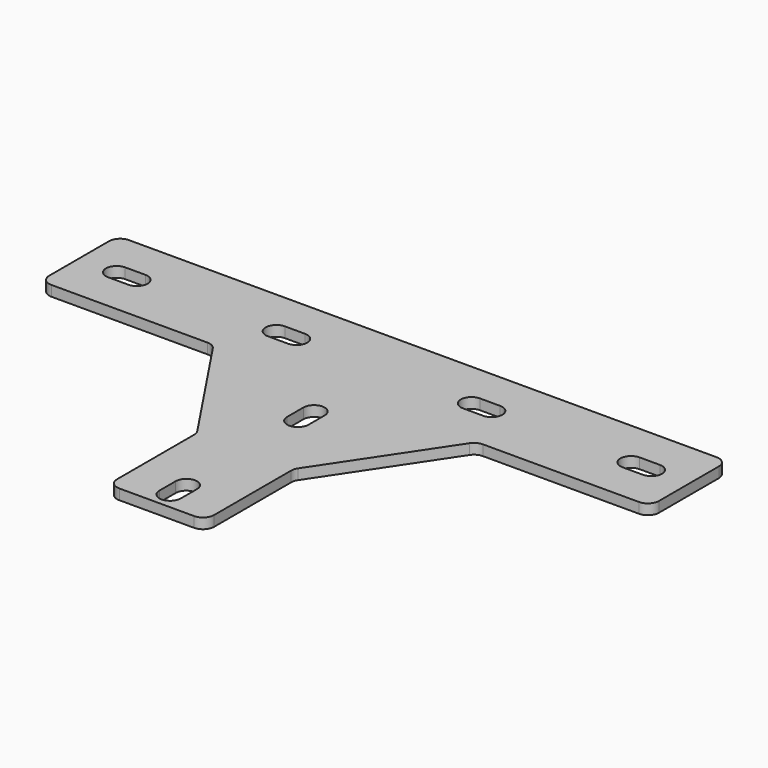
from build123d import *

# Parameters (mm, degrees)
F1_DEPTH = 4.7625
F2_R     = 5.08
F4_DEPTH = 4.7635


# Not quite as in the source:
# - a length typed as a fraction of an inch, garbled in the dataset ("3 / 203.2 mm" for 3/8 in), is restored


with BuildPart() as f1:
    # F0 (on Top) → F1 (new body)
    with BuildSketch(Plane.XY):
        Polygon((124.0544550598, 72.092982788), (-155.3455449402, 72.092982788), (-155.3455449402, 27.642982788), (-76.0003953454, 27.642982788), (-37.8705449402, -29.507017212), (-37.8705449402, -80.307017212), (6.5794550598, -80.307017212), (6.5794550598, -29.507017212), (44.7093054649, 27.642982788), (124.0544550598, 27.642982788), align=None)
    extrude(amount=F1_DEPTH)

    # F2
    f2_edges = [f1.edges().sort_by_distance(p)[0] for p in [
        (-155.345545, 27.642983, 2.38125),
        (-155.345545, 72.092983, 2.38125),
        (-37.870545, -80.307017, 2.38125),
        (6.579455, -80.307017, 2.38125),
        (-76.000395, 27.642983, 2.38125),
        (-37.870545, -29.507017, 2.38125),
        (6.579455, -29.507017, 2.38125),
        (44.709305, 27.642983, 2.38125),
        (124.054455, 27.642983, 2.38125),
        (124.054455, 72.092983, 2.38125),
    ]]
    fillet(f2_edges, radius=F2_R)

    # F3 (on face) → F4 (cut, through all)
    with BuildSketch(Plane.XY.offset(4.7625)):
        with BuildLine():
            Line((106.8459550598, 54.757482788), (97.5749550598, 54.757482788))
            ThreePointArc((97.5749550598, 54.757482788), (92.6854550598, 49.867982788), (97.5749550598, 44.978482788))
            Line((97.5749550598, 44.978482788), (106.8459550598, 44.978482788))
            ThreePointArc((106.8459550598, 44.978482788), (111.7354550598, 49.867982788), (106.8459550598, 54.757482788))
        make_face()
        with BuildLine():
            Line((33.6939550598, 54.757482788), (24.4229550598, 54.757482788))
            ThreePointArc((24.4229550598, 54.757482788), (19.5334550598, 49.867982788), (24.4229550598, 44.978482788))
            Line((24.4229550598, 44.978482788), (33.6939550598, 44.978482788))
            ThreePointArc((33.6939550598, 44.978482788), (38.5834550598, 49.867982788), (33.6939550598, 54.757482788))
        make_face()
        with BuildLine():
            ThreePointArc((-10.7560449402, -63.352517212), (-15.6455449402, -58.463017212), (-20.5350449402, -63.352517212))
            Line((-20.5350449402, -63.352517212), (-20.5350449402, -72.623517212))
            ThreePointArc((-20.5350449402, -72.623517212), (-15.6455449402, -77.513017212), (-10.7560449402, -72.623517212))
            Line((-10.7560449402, -72.623517212), (-10.7560449402, -63.352517212))
        make_face()
        with BuildLine():
            Line((-10.7560449402, 0.528482788), (-10.7560449402, 9.799482788))
            ThreePointArc((-10.7560449402, 9.799482788), (-15.6455449402, 14.688982788), (-20.5350449402, 9.799482788))
            Line((-20.5350449402, 9.799482788), (-20.5350449402, 0.528482788))
            ThreePointArc((-20.5350449402, 0.528482788), (-15.6455449402, -4.361017212), (-10.7560449402, 0.528482788))
        make_face()
        with BuildLine():
            Line((-128.8660449402, 54.757482788), (-138.1370449402, 54.757482788))
            ThreePointArc((-138.1370449402, 54.757482788), (-143.0265449402, 49.867982788), (-138.1370449402, 44.978482788))
            Line((-138.1370449402, 44.978482788), (-128.8660449402, 44.978482788))
            ThreePointArc((-128.8660449402, 44.978482788), (-123.9765449402, 49.867982788), (-128.8660449402, 54.757482788))
        make_face()
        with BuildLine():
            Line((-55.7140449402, 54.757482788), (-64.9850449402, 54.757482788))
            ThreePointArc((-64.9850449402, 54.757482788), (-69.8745449402, 49.867982788), (-64.9850449402, 44.978482788))
            Line((-64.9850449402, 44.978482788), (-55.7140449402, 44.978482788))
            ThreePointArc((-55.7140449402, 44.978482788), (-50.8245449402, 49.867982788), (-55.7140449402, 54.757482788))
        make_face()
    extrude(amount=-F4_DEPTH, mode=Mode.SUBTRACT)


solid = f1.part
